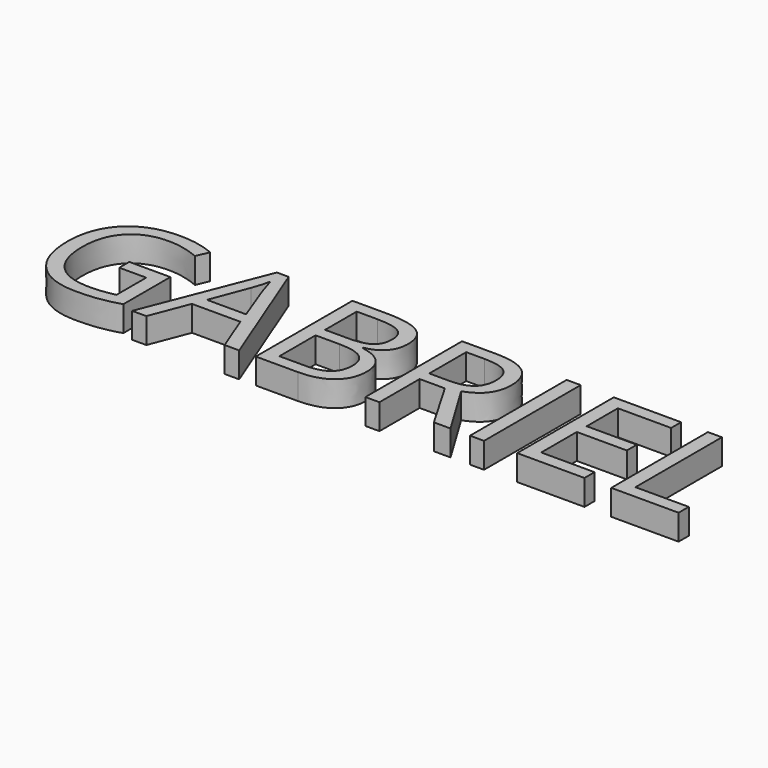
from build123d import *

# Parameters (mm, degrees)
F0_TEXT_SIZE = 49.8599683245
F1_DEPTH     = 7.5125228614


# Not quite as in the source:
# - Text() gives the source's letters only with a copy of the font that has no kerning and outlines rounded to 1/6400 em; it was checked with that copy


with BuildPart() as f1:
    # F0 (on Top) → F1 (new body)
    with BuildSketch(Plane.XY):
        with Locations((34.1297835112, 0)):
            Text('GABRIEL', F0_TEXT_SIZE, font='Open Sans', text_align=(TextAlign.LEFT, TextAlign.BOTTOM))
    extrude(amount=F1_DEPTH)


solid = f1.part
